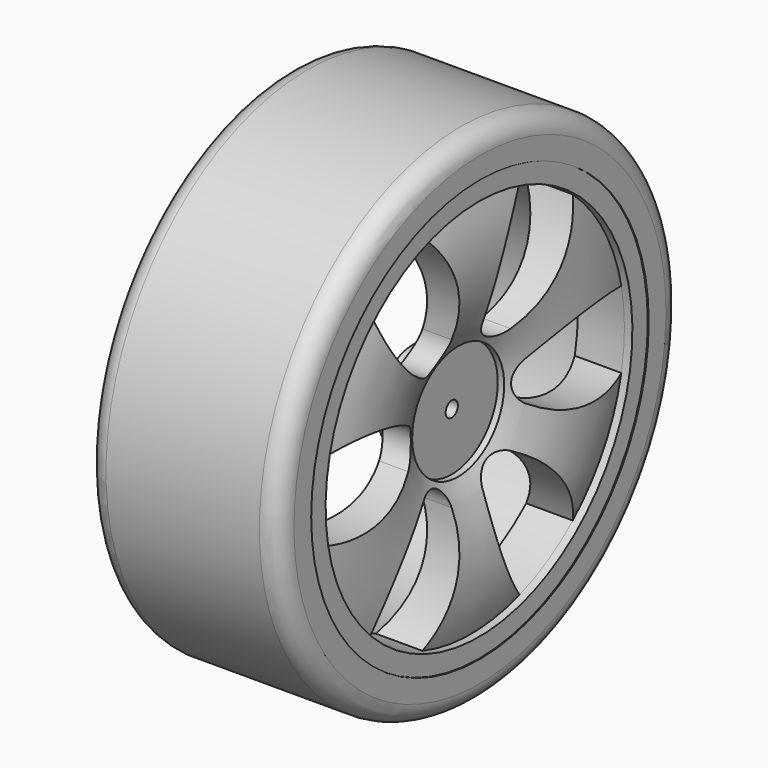
from build123d import *

# Parameters (mm, degrees)
F2_R            = 4
F4_DEPTH        = 40.001
F4_COPIES_COUNT = 6


# Not quite as in the source:
# - a pattern or mirror of a feature is missing from the dataset's text; its kind, count and spacing are read off the source's solid


with BuildPart() as f1:
    # F0 (on Front) → F1 (revolve)
    with BuildSketch(Plane.XZ):
        with BuildLine():
            Line((40, 52.5), (0, 52.5))
            Line((0, 52.5), (0, 40.5))
            Line((0, 40.5), (28.1262126109, 40.5))
            ThreePointArc((28.1262126109, 40.5), (32.616652359, 24.8422473669), (28.1262126109, 9.1844947338))
            Line((28.1262126109, 9.1844947338), (26, 9.1844947338))
            Line((26, 9.1844947338), (26, 5.4136281833))
            Line((26, 5.4136281833), (30.0027634948, 5.4136281833))
            Line((30.0027634948, 5.4136281833), (30.0027634948, 1.6))
            Line((30.0027634948, 1.6), (34.1176193349, 1.6))
            Line((34.1176193349, 1.6), (34.1176193349, 12))
            Line((34.1176193349, 12), (35.454442556, 12))
            ThreePointArc((35.454442556, 12), (39.7334179347, 25.718427341), (38.1391904146, 40))
            Line((38.1391904146, 40), (39.8, 40))
            Line((39.8, 40), (39.8, 44))
            Line((39.8, 44), (40, 44))
            Line((40, 44), (40, 52.5))
        make_face()
    revolve(axis=Axis((5.8233812451, 0, 0), (1, 0, 0)))

    # F2
    f2_edges = [f1.edges().sort_by_distance(p)[0] for p in [
        (40, 0, -52.5),
        (0, 0, -52.5),
    ]]
    fillet(f2_edges, radius=F2_R)

    # F3 (on face) → F4 (cut, through all)
    with BuildSketch(Plane.YZ.offset(40)):
        with BuildLine():
            ThreePointArc((12.667714712, 37.941125497), (5.9914990832, 27.5820805267), (4.0433834031, 15.4130003185))
            ThreePointArc((4.0433834031, 15.4130003185), (6.5375926866, 11.3234426924), (11.3263581228, 11.2081729036))
            ThreePointArc((11.3263581228, 11.2081729036), (20.8910328838, 18.9798306762), (26.5241211725, 29.941125497))
            ThreePointArc((26.5241211725, 29.941125497), (20, 34.6410161514), (12.667714712, 37.941125497))
        make_face()
    f4 = extrude(amount=-F4_DEPTH, mode=Mode.SUBTRACT)

    # F4_copies: F4 ×6 about axis
    f4_copies_axis = Axis((0, 0, 0), (1, 0, 0))
    for i in range(1, F4_COPIES_COUNT):
        add(f4.rotate(f4_copies_axis, i * 360 / F4_COPIES_COUNT), mode=Mode.SUBTRACT)


solid = f1.part
